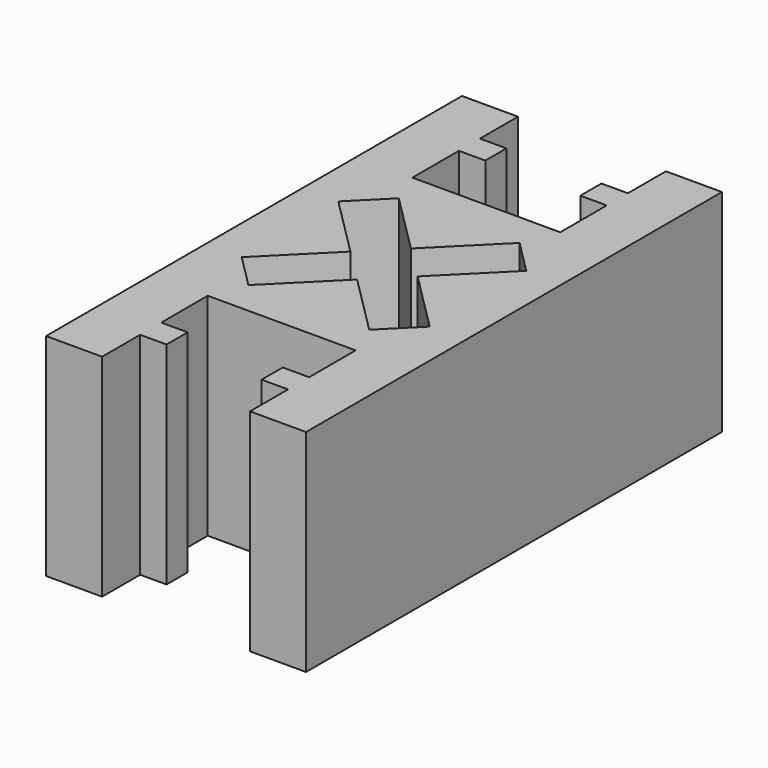
from build123d import *

# Parameters (mm, degrees)
F0_W             = 12.5
F0_H             = 25
F1_DEPTH         = 10.16
F2_W             = 7.112
F2_H             = 6.35
F3_DEPTH         = 25.4
F4_W             = 1.27
F4_H             = 1.27
F5_DEPTH         = 10.16
F5_COPIES2_COUNT = 2
F5_COPIES2_PITCH = 20.028927
F8_DEPTH         = 25.4


# Not quite as in the source:
# - a pattern or mirror of a feature is missing from the dataset's text; its kind, count and spacing are read off the source's solid


with BuildPart() as f1:
    # F0 (on Top) → F1 (new body)
    with BuildSketch(Plane.XY):
        Rectangle(F0_W, F0_H)
    extrude(amount=F1_DEPTH)

    # F2 (on face) → F3 (cut)
    with BuildSketch(Plane.XY.offset(10.16)):
        with Locations((0, -9.325)):
            Rectangle(F2_W, F2_H)
    f3 = extrude(amount=-F3_DEPTH, mode=Mode.SUBTRACT)

    # F3_copies: F3 across plane
    add(f3.mirror(Plane.ZX), mode=Mode.SUBTRACT)

    # F4 (on face) → F5 (join, through all)
    with BuildSketch(Plane.XY.offset(10.16)):
        with Locations((-2.921, -9.579)):
            Rectangle(F4_W, F4_H)
    f5 = extrude(amount=-F5_DEPTH)

    # F5_copies: F5 across plane
    add(f5.mirror(Plane(origin=(0, 0, 0), x_dir=(0, 0, 1), z_dir=(1, 0, 0))))

    # F5_copies1: F5 across plane
    add(f5.mirror(Plane.ZX))

    # F5_copies2: F5 ×2
    with Locations(*[Vector(0.2916781273, 0.9565165289, 0) * (i * F5_COPIES2_PITCH) for i in range(1, F5_COPIES2_COUNT)]):
        add(f5)

    # F7 (on face) → F8 (cut)
    with BuildSketch(Plane.XY.offset(10.16)):
        Polygon((-0.8082230509, 0.8082230509), (-4.5205336521, -2.9040875503), (-3.7123106012, -3.7123106012), (0, 0), align=None)
        Polygon((2.9040875503, 4.5205336521), (-0.8082230509, 0.8082230509), (0, 0), (-3.7123106012, -3.7123106012), (-2.9040875503, -4.5205336521), (4.5205336521, 2.9040875503), align=None)
    f8 = extrude(amount=-F8_DEPTH, mode=Mode.SUBTRACT)

    # F8_copies: F8 across plane
    add(f8.mirror(Plane(origin=(0, 0, 0), x_dir=(0, 0, 1), z_dir=(1, 0, 0))), mode=Mode.SUBTRACT)


solid = f1.part
